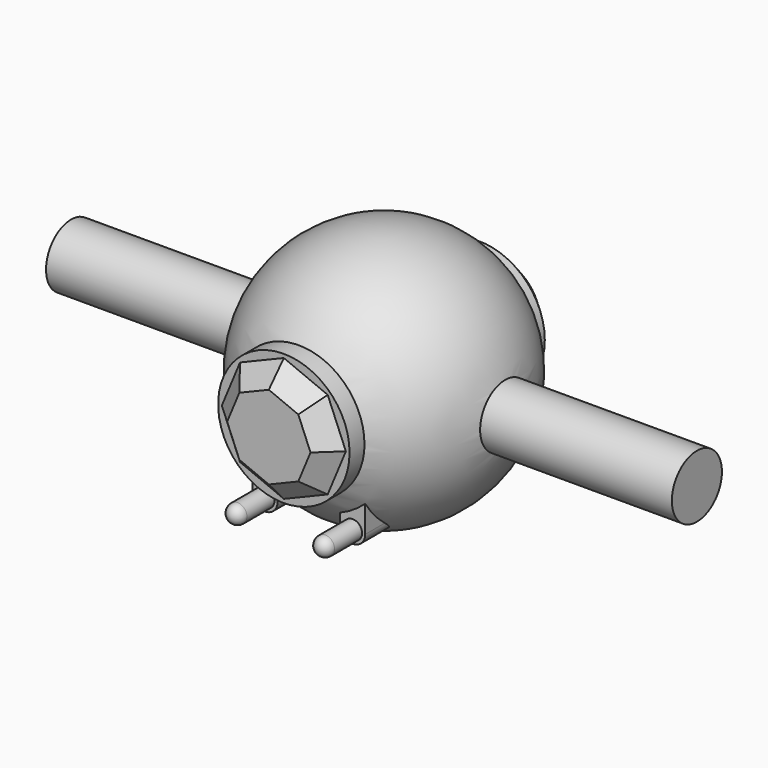
from build123d import *

# Parameters (mm, degrees)
F3_DEPTH  = 23
F4_SIZE   = 3
F5_R      = 10.5
F6_DEPTH  = 20
F7_R      = 10.5
F8_DEPTH  = 23
F9_SIZE   = 4
F11_R     = 1
F12_D     = 11
F12_DEPTH = 10
F12_TIP   = 3.3047334047
F13_R     = 5.5
F14_DEPTH = 15
F16_DEPTH = 1
F17_DEPTH = 7
F18_W     = 4
F18_H     = 7
F19_DEPTH = 15
F20_R     = 1.9999
F21_R     = 1.5
F22_DEPTH = 7
F23_R     = 1.5
F24_R     = 5
F25_DEPTH = 50


# Not quite as in the source:
# - a fillet or chamfer is up to 0.001 mm smaller than in the source, because OpenCascade refuses the exact size


with BuildPart() as f1:
    # F0 (on Front) → F1 (revolve)
    with BuildSketch(Plane.XZ):
        with BuildLine():
            Line((0, 15), (0, 20))
            ThreePointArc((0, 20), (-20, 0), (0, -20))
            Line((0, -20), (0, -15))
            ThreePointArc((0, -15), (-15, 0), (0, 15))
        make_face()
    revolve(axis=Axis((0, 0, 17.5), (0, 0, -1)))

    # F2 (on Front) → F3 (join)
    with BuildSketch(Plane.XZ):
        Polygon((-3.293e-07, -9.9083022872), (7.0062275045, -7.0062279701), (9.9083022872, -3.293e-07), (7.0062279701, 7.0062275045), (3.293e-07, 9.9083022872), (-7.0062275045, 7.0062279701), (-9.9083022872, 3.293e-07), (-7.0062279701, -7.0062275045), align=None)
    extrude(amount=F3_DEPTH)

    # F4
    f4_edges = [f1.edges().sort_by_distance(p)[0] for p in [
        (-3.503114, -23, 8.457265),
        (3.503114, -23, 8.457265),
        (-8.457265, -23, 3.503114),
        (-8.457265, -23, -3.503114),
        (-3.503114, -23, -8.457265),
        (3.503114, -23, -8.457265),
        (8.457265, -23, -3.503114),
        (8.457265, -23, 3.503114),
    ]]
    chamfer(f4_edges, length=F4_SIZE)

    # F5 (on Front) → F6 (join)
    with BuildSketch(Plane.XZ):
        Circle(F5_R)
    extrude(amount=F6_DEPTH)

    # F7 (on Front) → F8 (join)
    with BuildSketch(Plane.XZ):
        Circle(F7_R)
    extrude(amount=-F8_DEPTH)

    # F9
    f9_edges = [f1.edges().sort_by_distance(p)[0] for p in [
        (-10.5, 23, 0),
    ]]
    chamfer(f9_edges, length=F9_SIZE)

    # F11
    f11_edges = [f1.edges().sort_by_distance(p)[0] for p in [
        (-6.5, 23, 0),
    ]]
    fillet(f11_edges, radius=F11_R)

    # F12
    with Locations(Plane(origin=(0, 23, 0), x_dir=(-1, 0, 0), z_dir=(0, 1, 0))):
        with Locations((0, 0)):
            Hole(F12_D / 2, depth=F12_DEPTH)
            with Locations((0, 0, -(F12_DEPTH + F12_TIP / 2))):  # 118° drill point
                Cone(0, F12_D / 2, F12_TIP, mode=Mode.SUBTRACT)

    # F13 (on Front) → F14 (join)
    with BuildSketch(Plane.XZ):
        Circle(F13_R)
    extrude(amount=-F14_DEPTH)

    # F15 (on face) → F16 (join)
    with BuildSketch(Plane(origin=(0, 15, 0), x_dir=(-1, 0, 0), z_dir=(0, 1, 0))):
        Polygon((0, 2.6071637132), (-4.249590449, 1.3460217891), (-4.249590449, -1.4039782109), (0, -2.3928362868), (4.250409551, -1.4039782109), (4.250409551, 1.3460217891), align=None)
    extrude(amount=F16_DEPTH)

    # F17 (cut): a face of the model
    f17_faces = [f1.faces().sort_by_distance(p)[0] for p in [
        (-0.000369917, 16, 0.0456802636),
    ]]
    extrude(f17_faces, amount=-F17_DEPTH, mode=Mode.SUBTRACT)

    # F18 (on Front) → F19 (join)
    with BuildSketch(Plane.XZ):
        with Locations((-7, -12.5)):
            Rectangle(F18_W, F18_H)
        with Locations((7, -12.5)):
            Rectangle(F18_W, F18_H)
    extrude(amount=F19_DEPTH)

    # F20 (radius 2 in the source; OpenCascade refuses exactly that, so slightly less here)
    f20_edges = [f1.edges().sort_by_distance(p)[0] for p in [
        (-9, -11.468627, -16),
        (-5, -12.954356, -16),
        (5, -12.954356, -16),
        (9, -11.468627, -16),
    ]]
    fillet(f20_edges, radius=F20_R)

    # F21 (on face) → F22 (join)
    with BuildSketch(Plane.XZ.offset(15)):
        with Locations((-7, -14)):
            Circle(F21_R)
        with Locations((7, -14)):
            Circle(F21_R)
    extrude(amount=F22_DEPTH)

    # F23
    f23_edges = [f1.edges().sort_by_distance(p)[0] for p in [
        (-8.5, -22, -14),
        (5.5, -22, -14),
    ]]
    fillet(f23_edges, radius=F23_R)

    # F24 (on Right) → F25 (join, symmetric)
    with BuildSketch(Plane.YZ):
        Circle(F24_R)
    extrude(amount=F25_DEPTH, both=True)


solid = f1.part
